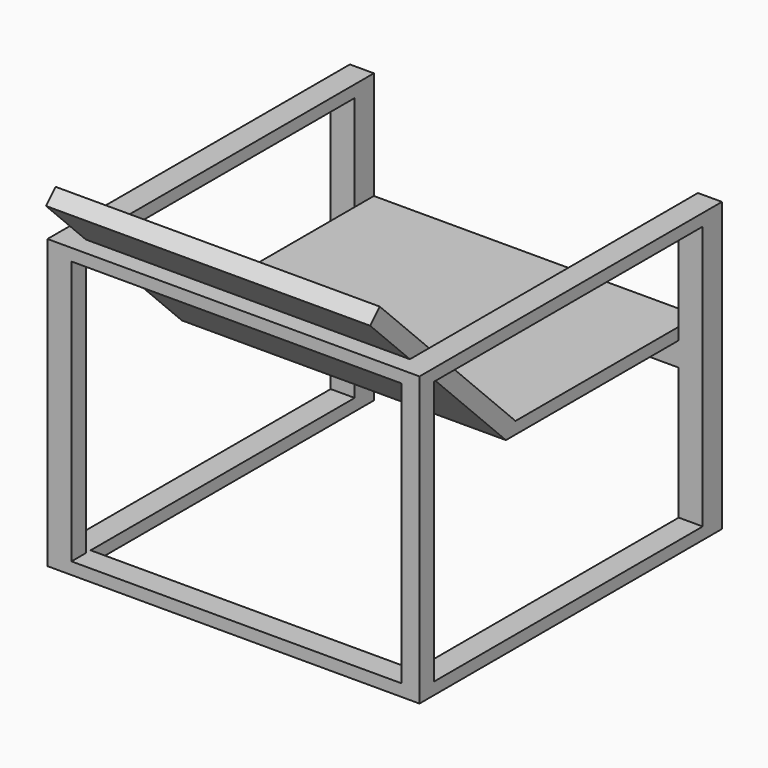
from build123d import *

# Parameters (mm, degrees)
F0_W      = 787.4
F0_H      = 50.8
F1_DEPTH  = 609.6
F2_W      = 711.2
F2_H      = 558.8
F3_DEPTH  = 50.8
F4_W      = 38.1
F4_H      = 609.6
F5_DEPTH  = 736.6
F6_W      = 711.2
F6_H      = 558.8
F7_DEPTH  = 50.8
F8_DEPTH  = 12.7
F10_DEPTH = 736.6
F11_DEPTH = 12.7
F12_W     = 711.2
F12_H     = 558.8
F13_DEPTH = 50.8
F14_W     = 38.1
F14_H     = 50.8
F15_DEPTH = 711.2
F16_DEPTH = 12.7
F17_W     = 685.8
F17_H     = 508
F18_DEPTH = 25.4
F19_SIZE  = 25.39999
F20_W     = 685.8
F20_H     = 35.9210244843
F21_DEPTH = 508


# Not quite as in the source:
# - a fillet or chamfer is up to 0.001 mm smaller than in the source, because OpenCascade refuses the exact size


with BuildPart() as f1:
    # F0 (on Top) → F1 (new body)
    with BuildSketch(Plane.XY):
        with Locations((273.7565302372, -36.9653456569)):
            Rectangle(F0_W, F0_H)
    extrude(amount=F1_DEPTH)

    # F2 (on face) → F3 (cut)
    with BuildSketch(Plane.XZ.offset(62.3653456569)):
        with Locations((273.7565302372, 304.8)):
            Rectangle(F2_W, F2_H)
    extrude(amount=-F3_DEPTH, mode=Mode.SUBTRACT)

    # F4 (on face) → F5 (join)
    with BuildSketch(Plane(origin=(0, -11.5653456569, 0), x_dir=(-1, 0, 0), z_dir=(0, 1, 0))):
        with Locations((-648.4065302372, 304.8)):
            Rectangle(F4_W, F4_H)
    extrude(amount=F5_DEPTH)

    # F6 (on face) → F7 (cut)
    with BuildSketch(Plane.YZ.offset(667.4565302372)):
        with Locations((331.3346543431, 304.8)):
            Rectangle(F6_W, F6_H)
    extrude(amount=-F7_DEPTH, mode=Mode.SUBTRACT)

    # F8 (add): a face of the model
    f8_faces = [f1.faces().sort_by_distance(p)[0] for p in [
        (629.3565302372, -2.0040083027, 12.7),
    ]]
    extrude(f8_faces, amount=F8_DEPTH)

    # F9 (on face) → F10 (join)
    with BuildSketch(Plane(origin=(0, -11.5653456569, 0), x_dir=(-1, 0, 0), z_dir=(0, 1, 0))):
        Polygon((119.9434697628, 0), (119.9434697628, 609.6), (81.8434697628, 609.6), (81.8434697628, 584.2), (81.8434697628, 25.4), (81.8434697628, 0), align=None)
    extrude(amount=F10_DEPTH)

    # F11 (add): a face of the model
    f11_faces = [f1.faces().sort_by_distance(p)[0] for p in [
        (-81.8434697628, 333.3254651539, 304.8),
    ]]
    extrude(f11_faces, amount=F11_DEPTH)

    # F12 (on face) → F13 (cut)
    with BuildSketch(Plane(origin=(-119.9434697628, 0, 0), x_dir=(0, -1, 0), z_dir=(-1, 0, 0))):
        with Locations((-331.3346543431, 304.8)):
            Rectangle(F12_W, F12_H)
    extrude(amount=-F13_DEPTH, mode=Mode.SUBTRACT)

    # F14 (on face) → F15 (join)
    with BuildSketch(Plane.YZ.offset(-69.1434697628)):
        with Locations((705.9846543431, 330.2)):
            Rectangle(F14_W, F14_H)
    extrude(amount=F15_DEPTH)

    # F16 (add): a face of the model
    f16_faces = [f1.faces().sort_by_distance(p)[0] for p in [
        (273.7565302372, 725.0346543431, 313.944),
    ]]
    extrude(f16_faces, amount=F16_DEPTH)

    # F17 (on face) → F18 (join)
    with BuildSketch(Plane.XY.offset(355.6)):
        with Locations((273.7565302372, 483.7346543431)):
            Rectangle(F17_W, F17_H)
    extrude(amount=F18_DEPTH)

    # F19 (size 25.4 in the source; OpenCascade refuses exactly that, so slightly less here)
    f19_edges = [f1.edges().sort_by_distance(p)[0] for p in [
        (273.75653, 229.734654, 381),
    ]]
    chamfer(f19_edges, length=F19_SIZE)

    # F20 (on face) → F21 (join)
    with BuildSketch(Plane(origin=(0, -62.9326728284, 62.9326728284), x_dir=(1, 0, 0), z_dir=(0, -0.7071067812, 0.7071067812))):
        with Locations((273.7565302372, 431.8546155916)):
            Rectangle(F20_W, F20_H)
    extrude(amount=F21_DEPTH)


solid = f1.part
